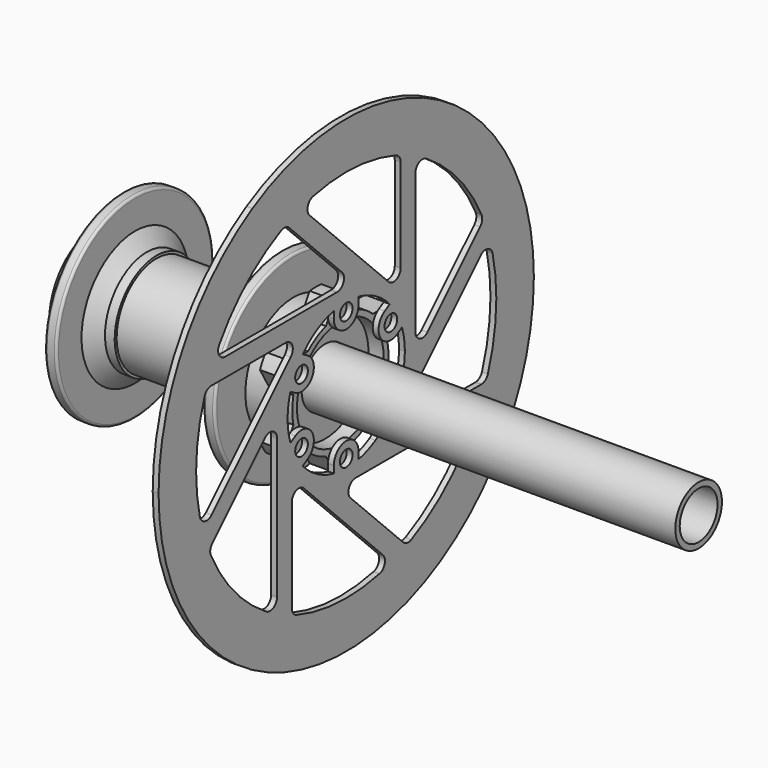
from build123d import *

# Parameters (mm, degrees)
F2_SIZE2       = 4
F2_SIZE        = 5
F3_R           = 0.8
F5_R           = 20.5
F6_DEPTH       = 16
F8_DEPTH       = 8.5
F9_COUNT       = 6
F10_R          = 18.5
F11_DEPTH      = 14.2
F12_DEPTH      = 9
F13_R          = 22
F14_DEPTH      = 9
F14_TAPER      = 10
F15_R          = 18.5
F16_DEPTH      = 14.2
F17_DEPTH      = 9
F18_R          = 10
F19_DEPTH      = 38.0010001
F19_DEPTH_BACK = 45.001
F20_R          = 2.7
F21_DEPTH      = 2
F22_COUNT      = 6
F24_DEPTH      = 85.0010001
F25_COUNT      = 8
F26_R          = 9.95
F26_R_2        = 8.0645
F27_DEPTH      = 200


with BuildPart() as f1:
    # F0 (on Front) → F1 (revolve)
    with BuildSketch(Plane.XZ):
        Polygon((0, 17), (0, 0), (29, 0), (29, 33.5), (25, 33.5), (25, 17.85), (17.7, 17.85), (17.7, 17), align=None)
    revolve(axis=Axis((-10.4847326972, 0, 0), (-1, 0, 0)))

    # F2
    f2_edges = [f1.edges().sort_by_distance(p)[0] for p in [
        (25, 0, -17.85),
    ]]
    chamfer(f2_edges, length=F2_SIZE, length2=F2_SIZE2)

    # F3
    f3_edges = [f1.edges().sort_by_distance(p)[0] for p in [
        (25, 0, -33.5),
        (29, 0, -33.5),
    ]]
    fillet(f3_edges, radius=F3_R)

    # F4: F1 across face


with BuildPart() as f1_1:
    add(f1.part)
    add(f1.part.mirror(Plane(origin=(0, 0, 0), x_dir=(0, -1, 0), z_dir=(-1, 0, 0))))

    # F5 (on face) → F6 (join)
    with BuildSketch(Plane.YZ.offset(29)):
        Circle(F5_R)
    extrude(amount=F6_DEPTH)

    # F7 (on face) → F8 (join)
    with BuildSketch(Plane.YZ.offset(45)):
        with BuildLine():
            Line((17.4415527975, 0), (2.5, 25.8795285892))
            ThreePointArc((2.5, 25.8795285892), (0, 26), (-2.5, 25.8795285892))
            Line((-2.5, 25.8795285892), (-17.4415527975, 0))
            Line((-17.4415527975, 0), (17.4415527975, 0))
        make_face()
    f8 = extrude(amount=-F8_DEPTH)

    # F9: F8 ×6 about axis
    f9_axis = Axis((14.5, 0, 0), (1, 0, 0))
    for i in range(1, F9_COUNT):
        add(f8.rotate(f9_axis, i * 360 / F9_COUNT))

    # F10 (on face) → F11 (cut)
    with BuildSketch(Plane.YZ.offset(45)):
        Circle(F10_R)
    extrude(amount=-F11_DEPTH, mode=Mode.SUBTRACT)


with BuildPart() as f12:
    # F12 (new): a face of the model
    f12_faces = [f1_1.part.faces().sort_by_distance(p)[0] for p in [
        (30.8, 0, 0),
    ]]
    extrude(f12_faces, amount=F12_DEPTH)


with BuildPart() as f1_2:
    add(f1_1.part)

    # F13 (on face) → F14 (join)
    with BuildSketch(Plane(origin=(-29, 0, 0), x_dir=(0, -1, 0), z_dir=(-1, 0, 0))):
        Circle(F13_R)
    extrude(amount=F14_DEPTH, taper=F14_TAPER)

    # F15 (on face) → F16 (cut)
    with BuildSketch(Plane(origin=(-38, 0, 0), x_dir=(0, -1, 0), z_dir=(-1, 0, 0))):
        Circle(F15_R)
    extrude(amount=-F16_DEPTH, mode=Mode.SUBTRACT)


with BuildPart() as f17:
    # F17 (new): a face of the model
    f17_faces = [f1_2.part.faces().sort_by_distance(p)[0] for p in [
        (-23.8, 0, 0),
    ]]
    extrude(f17_faces, amount=F17_DEPTH)


with BuildPart() as f19_tool:
    # F18 (on Right) → F19 (new body, two sides)
    with BuildSketch(Plane.YZ) as f19_sk:
        Circle(F18_R)
    extrude(amount=-F19_DEPTH)
    extrude(f19_sk.sketch, amount=F19_DEPTH_BACK)


with BuildPart() as f1_3:
    add(f1_2.part)

    # F19: cut by f19_tool
    add(f19_tool.part, mode=Mode.SUBTRACT)


with BuildPart() as f12_1:
    add(f12.part)

    # F19: cut by f19_tool
    add(f19_tool.part, mode=Mode.SUBTRACT)


with BuildPart() as f17_1:
    add(f17.part)

    # F19: cut by f19_tool
    add(f19_tool.part, mode=Mode.SUBTRACT)


with BuildPart() as f21:
    # F20 (on face) → F21 (new body)
    with BuildSketch(Plane.YZ.offset(45)):
        with BuildLine():
            ThreePointArc((-12.5, 21.6506350946), (-8.9841138004, 23.329931402), (-5.25, 24.4425346476))
            Line((-5.25, 24.4425346476), (-5.25, 22))
            ThreePointArc((-5.25, 22), (0, 16.75), (5.25, 22))
            Line((5.25, 22), (5.25, 24.4425346476))
            ThreePointArc((5.25, 24.4425346476), (8.9841138004, 23.329931402), (12.5, 21.6506350946))
            Line((12.5, 21.6506350946), (40, 69.2820323028))
            ThreePointArc((40, 69.2820323028), (0, 80), (-40, 69.2820323028))
            Line((-40, 69.2820323028), (-12.5, 21.6506350946))
        make_face()
        with Locations((0, 22)):
            Circle(F20_R, mode=Mode.SUBTRACT)
    extrude(amount=F21_DEPTH)

    # F22: F21 ×6 about axis
    f22_axis = Axis((14.5, 0, 0), (1, 0, 0))


with BuildPart() as f21_1:
    add(f21.part)
    for i in range(1, F22_COUNT):
        add(f21.part.rotate(f22_axis, i * 360 / F22_COUNT))

    # F23 (on face) → F24 (cut, through all)
    with BuildSketch(Plane.YZ.offset(47)):
        with BuildLine():
            ThreePointArc((-54.1599649242, 34.0983606557), (-54.2475335682, 31.0500141323), (-51.6212165684, 29.5))
            Line((-51.6212165684, 29.5), (-3.9328860401, 29.5))
            ThreePointArc((-3.9328860401, 29.5), (-1.1612474425, 31.3519497029), (-1.8115656965, 34.6213203436))
            Line((-1.8115656965, 34.6213203436), (-24.2949998262, 57.1047544732))
            ThreePointArc((-24.2949998262, 57.1047544732), (-25.9124406651, 57.940815648), (-27.7154834568, 57.6875374475))
            ThreePointArc((-27.7154834568, 57.6875374475), (-42.6029292106, 47.7597154794), (-54.1599649242, 34.0983606557))
        make_face()
    f24 = extrude(amount=-F24_DEPTH, mode=Mode.SUBTRACT)

    # F25: F24 ×8 about axis
    f25_axis = Axis((14.5, 0, 0), (1, 0, 0))
    for i in range(1, F25_COUNT):
        add(f24.rotate(f25_axis, i * 360 / F25_COUNT), mode=Mode.SUBTRACT)


with BuildPart() as f27:
    # F26 (on face) → F27 (new body)
    with BuildSketch(Plane(origin=(-32.8, 0, 0), x_dir=(0, -1, 0), z_dir=(-1, 0, 0))):
        Circle(F26_R)
        Circle(F26_R_2, mode=Mode.SUBTRACT)
    extrude(amount=-F27_DEPTH)


solid = Compound([f1_3.part, f12_1.part, f17_1.part, f21_1.part, f27.part])
